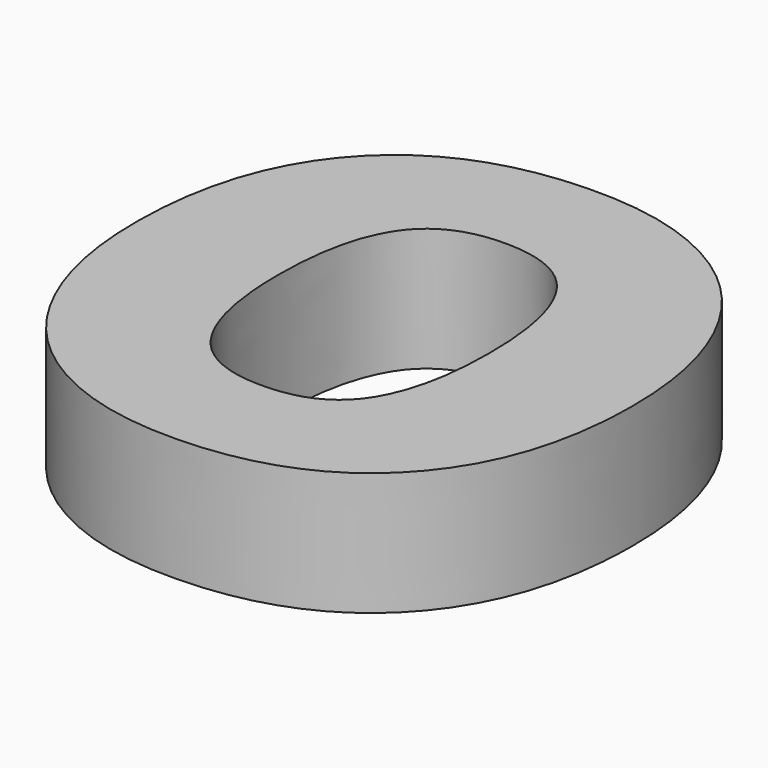
from build123d import *

# Parameters (mm, degrees)
F0_TEXT_SIZE = 76.2947990249
F1_DEPTH     = 10


# Not quite as in the source:
# - Text() gives the source's letters only with a copy of the font that has no kerning and outlines rounded to 1/6400 em; it was checked with that copy


with BuildPart() as f1:
    # F0 (on Top) → F1 (new body)
    with BuildSketch(Plane.XY):
        with Locations((0, 0)):
            Text('o', F0_TEXT_SIZE, font='Open Sans', font_style=FontStyle.BOLD, text_align=(TextAlign.LEFT, TextAlign.BOTTOM))
    extrude(amount=F1_DEPTH)


solid = f1.part
